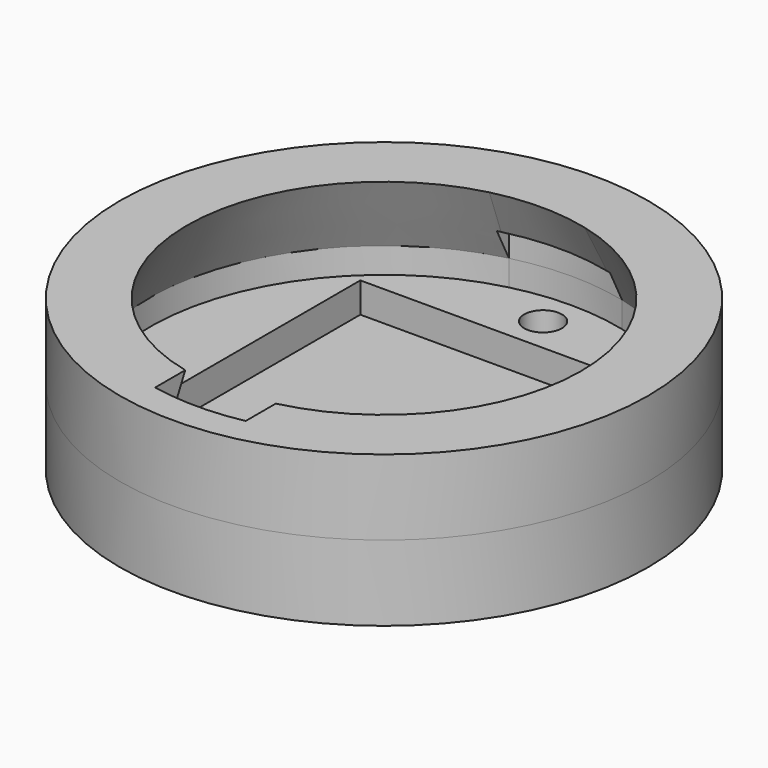
from build123d import *

# Parameters (mm, degrees)
F0_R      = 35
F1_DEPTH  = 10
F2_R      = 2.5
F3_DEPTH  = 3.4
F4_DEPTH  = 10.001
F5_DEPTH  = 7.4
F2_R_2    = 35
F6_DEPTH  = 10
F6_TAPER  = -26
F7_R      = 39.8773258857
F7_R_2    = 35
F8_DEPTH  = 20.001
F9_DEPTH  = 4
F10_DEPTH = 10.0010001


# Not quite as in the source:
# - a feature names something its author has since deleted; it is built from what else it names


with BuildPart() as f1:
    # F0 (on Top) → F1 (new body)
    with BuildSketch(Plane.XY):
        Circle(F0_R)
    extrude(amount=F1_DEPTH)

    # F2 (on face) → F3 (cut)
    with BuildSketch(Plane.XY.offset(10)):
        with BuildLine():
            Line((7.5, 21.7), (7.5, 30.0790624854))
            ThreePointArc((7.5, 30.0790624854), (0, 31), (-7.5, 30.0790624854))
            Line((-7.5, 30.0790624854), (-7.5, 21.7))
            Line((-7.5, 21.7), (7.5, 21.7))
        make_face()
        with Locations((0, 26.35)):
            Circle(F2_R, mode=Mode.SUBTRACT)
        with BuildLine():
            Line((-7.5, 21.7), (-7.5, 30.0790624854))
            ThreePointArc((-7.5, 30.0790624854), (-30.9904741103, -0.7684493597), (-6, -30.4138126515))
            Line((-6, -30.4138126515), (-6, -21.7))
            Line((-6, -21.7), (-20.5, -21.7))
            Line((-20.5, -21.7), (-20.5, 21.7))
            Line((-20.5, 21.7), (-7.5, 21.7))
        make_face()
        with BuildLine():
            ThreePointArc((-6, -30.4138126515), (0, -31), (6, -30.4138126515))
            Line((6, -30.4138126515), (6, -21.7))
            Line((6, -21.7), (-6, -21.7))
            Line((-6, -21.7), (-6, -30.4138126515))
        make_face()
        with BuildLine():
            ThreePointArc((6, -30.4138126515), (23.9478600297, -19.685019685), (31, 0))
            ThreePointArc((31, 0), (24.4284670006, 19.085334684), (7.5, 30.0790624854))
            Line((7.5, 30.0790624854), (7.5, 21.7))
            Line((7.5, 21.7), (20.5, 21.7))
            Line((20.5, 21.7), (20.5, -21.7))
            Line((20.5, -21.7), (6, -21.7))
            Line((6, -21.7), (6, -30.4138126515))
        make_face()
    extrude(amount=-F3_DEPTH, mode=Mode.SUBTRACT)

    # F2 (on face) → F4 (cut, through all)
    with BuildSketch(Plane.XY.offset(10)):
        with Locations((0, 26.35)):
            Circle(F2_R)
    extrude(amount=-F4_DEPTH, mode=Mode.SUBTRACT)

    # F2 (on face) → F5 (cut)
    with BuildSketch(Plane.XY.offset(10)):
        Polygon((20.5, 21.7), (7.5, 21.7), (7.5, 20.0790624854), (0, 20.0790624854), (-7.5, 20.0790624854), (-7.5, 21.7), (-20.5, 21.7), (-20.5, -21.7), (-6, -21.7), (-6, -20.4138126515), (0, -20.4138126515), (6, -20.4138126515), (6, -21.7), (20.5, -21.7), align=None)
        Polygon((7.5, 20.0790624854), (7.5, 21.7), (-7.5, 21.7), (-7.5, 20.0790624854), (0, 20.0790624854), align=None)
        Polygon((-6, -21.7), (6, -21.7), (6, -20.4138126515), (0, -20.4138126515), (-6, -20.4138126515), align=None)
    extrude(amount=-F5_DEPTH, mode=Mode.SUBTRACT)

    # F2 (on face) → F6 (join)
    with BuildSketch(Plane.XY.offset(10)):
        Circle(F2_R_2)
        with BuildLine():
            ThreePointArc((7.5, 30.0790624854), (24.4284670006, 19.085334684), (31, 0))
            ThreePointArc((31, 0), (23.9478600297, -19.685019685), (6, -30.4138126515))
            ThreePointArc((6, -30.4138126515), (0, -31), (-6, -30.4138126515))
            ThreePointArc((-6, -30.4138126515), (-30.9904741103, -0.7684493597), (-7.5, 30.0790624854))
            ThreePointArc((-7.5, 30.0790624854), (0, 31), (7.5, 30.0790624854))
        make_face(mode=Mode.SUBTRACT)
    extrude(amount=F6_DEPTH, taper=F6_TAPER)

    # F7 (on face) → F8 (cut, through all)
    with BuildSketch(Plane.XY.offset(20)):
        Circle(F7_R)
        Circle(F7_R_2, mode=Mode.SUBTRACT)
    extrude(amount=-F8_DEPTH, mode=Mode.SUBTRACT)

    # F2 (on face) → F9 (cut)
    with BuildSketch(Plane.XY.offset(10)):
        with BuildLine():
            Line((7.5, 21.7), (7.5, 30.0790624854))
            ThreePointArc((7.5, 30.0790624854), (0, 31), (-7.5, 30.0790624854))
            Line((-7.5, 30.0790624854), (-7.5, 21.7))
            Line((-7.5, 21.7), (7.5, 21.7))
        make_face()
        with Locations((0, 26.35)):
            Circle(F2_R, mode=Mode.SUBTRACT)
        Polygon((7.5, 20.0790624854), (7.5, 21.7), (-7.5, 21.7), (-7.5, 20.0790624854), (0, 20.0790624854), align=None)
        with Locations((0, 26.35)):
            Circle(F2_R)
    extrude(amount=F9_DEPTH, mode=Mode.SUBTRACT)

    # F2 (on face) → F10 (cut, through all)
    with BuildSketch(Plane.XY.offset(10)):
        with BuildLine():
            ThreePointArc((-6, -30.4138126515), (0, -31), (6, -30.4138126515))
            Line((6, -30.4138126515), (6, -21.7))
            Line((6, -21.7), (-6, -21.7))
            Line((-6, -21.7), (-6, -30.4138126515))
        make_face()
        Polygon((-6, -21.7), (6, -21.7), (6, -20.4138126515), (0, -20.4138126515), (-6, -20.4138126515), align=None)
    extrude(amount=F10_DEPTH, mode=Mode.SUBTRACT)


solid = f1.part
